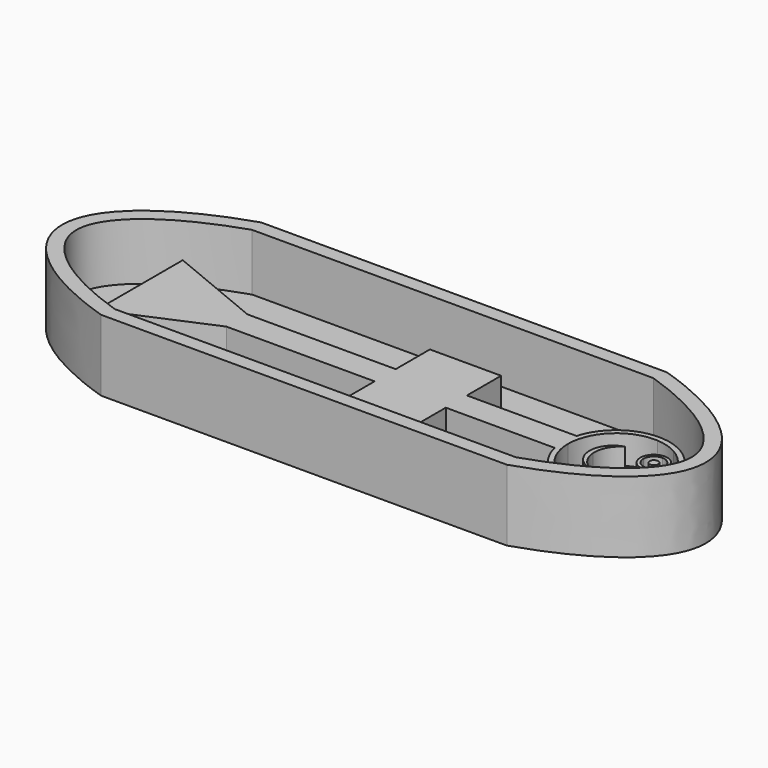
from build123d import *

# Parameters (mm, degrees)
F1_DEPTH  = 12.7
F2_T      = -2.54
F3_R      = 9.525
F4_DEPTH  = 5.08
F5_W      = 58.697837091
F5_H      = 4.7092778205
F6_DEPTH  = 5.08
F8_DEPTH  = 5.08
F9_W      = 12.7
F9_H      = 7.62
F10_DEPTH = 5.08


with BuildPart() as f1:
    # F0 (on Top) → F1 (new body)
    with BuildSketch(Plane.XY):
        with BuildLine():
            Line((-36.1903431505, -17.8440727383), (36.1903431505, -17.8440727383))
            add(Edge.make_bspline(
                [(36.1903431505, -17.8440727383), (91.0502120584, 0), (36.1903431505, 17.8440727383)],
                knots=[2.2529388906, 2.2529388906, 2.2529388906, 4.0302464165, 4.0302464165, 4.0302464165], degree=2, weights=[1, 0.6304575787, 1]))
            Line((36.1903431505, 17.8440727383), (-36.1903431505, 17.8440727383))
            add(Edge.make_bspline(
                [(-36.1903431505, 17.8440727383), (-91.0502120584, 0), (-36.1903431505, -17.8440727383)],
                knots=[5.3945315442, 5.3945315442, 5.3945315442, 7.1718390701, 7.1718390701, 7.1718390701], degree=2, weights=[1, 0.6304575787, 1]))
        make_face()
    extrude(amount=F1_DEPTH)

    # F2
    f2_openings = [f1.faces().sort_by_distance(p)[0] for p in [
        (0, 0, 12.7),
    ]]
    offset(amount=F2_T, openings=f2_openings, kind=Kind.INTERSECTION)

    # F3 (on face) → F4 (join)
    with BuildSketch(Plane.XY.offset(2.54)):
        with Locations((41.4168211738, 0)):
            Circle(F3_R)
        with BuildLine():
            ThreePointArc((49.4494469318, 3.058769096), (49.8702806957, 1.5550456789), (50.0121190134, 0))
            ThreePointArc((50.0121190134, 0), (49.8638586871, -1.5895603794), (49.4241923942, -3.1242840923))
            ThreePointArc((49.4241923942, -3.1242840923), (47.9319414134, -5.6064563866), (45.6999853593, -7.452090278))
            ThreePointArc((45.6999853593, -7.452090278), (43.8819573516, -8.2342120799), (41.9332322253, -8.57977066))
            ThreePointArc((41.9332322253, -8.57977066), (35.5244346388, -6.2577093152), (32.8215233342, 0))
            ThreePointArc((32.8215233342, 0), (35.5244346388, 6.2577093152), (41.9332322253, 8.57977066))
            ThreePointArc((41.9332322253, 8.57977066), (43.8819573516, 8.2342120799), (45.6999853593, 7.452090278))
            ThreePointArc((45.6999853593, 7.452090278), (47.9547863187, 5.5797989853), (49.4494469318, 3.058769096))
        make_face(mode=Mode.SUBTRACT)
        with BuildLine():
            Line((45.6999853593, 4.9295564949), (45.6999853593, 5.471769096))
            ThreePointArc((45.6999853593, 5.471769096), (43.9937366963, 4.765017759), (43.2869853593, 3.058769096))
            Line((43.2869853593, 3.058769096), (43.8291979604, 3.058769096))
            ThreePointArc((43.8291979604, 3.058769096), (44.3771389034, 4.381615552), (45.6999853593, 4.9295564949))
        make_face()
        with BuildLine():
            Line((47.5707727582, 3.058769096), (48.1129853593, 3.058769096))
            ThreePointArc((48.1129853593, 3.058769096), (47.4062340223, 4.765017759), (45.6999853593, 5.471769096))
            Line((45.6999853593, 5.471769096), (45.6999853593, 4.9295564949))
            ThreePointArc((45.6999853593, 4.9295564949), (47.0228318152, 4.381615552), (47.5707727582, 3.058769096))
        make_face()
        with BuildLine():
            ThreePointArc((45.6999853593, 0.645769096), (47.4062340223, 1.352520433), (48.1129853593, 3.058769096))
            Line((48.1129853593, 3.058769096), (47.5707727582, 3.058769096))
            ThreePointArc((47.5707727582, 3.058769096), (47.0228318152, 1.7359226401), (45.6999853593, 1.1879816971))
            Line((45.6999853593, 1.1879816971), (45.6999853593, 0.645769096))
        make_face()
        with BuildLine():
            ThreePointArc((43.2869853593, 3.058769096), (43.9937366963, 1.352520433), (45.6999853593, 0.645769096))
            Line((45.6999853593, 0.645769096), (45.6999853593, 1.1879816971))
            ThreePointArc((45.6999853593, 1.1879816971), (44.3771389034, 1.7359226401), (43.8291979604, 3.058769096))
            Line((43.8291979604, 3.058769096), (43.2869853593, 3.058769096))
        make_face()
        with BuildLine():
            Line((45.6999853593, -1.2536188461), (45.6999853593, -0.7113778659))
            ThreePointArc((45.6999853593, -0.7113778659), (43.9800014557, -1.4105307746), (43.2657123098, -3.1242840923))
            Line((43.2657123098, -3.1242840923), (43.8079261098, -3.1242840923))
            ThreePointArc((43.8079261098, -3.1242840923), (44.363409364, -1.7939385858), (45.6999853593, -1.2536188461))
        make_face()
        with BuildLine():
            ThreePointArc((43.2657123098, -3.1242840923), (43.9800014557, -4.8380374101), (45.6999853593, -5.5371903187))
            Line((45.6999853593, -5.5371903187), (45.6999853593, -4.9949493386))
            ThreePointArc((45.6999853593, -4.9949493386), (44.363409364, -4.4546295989), (43.8079261098, -3.1242840923))
            Line((43.8079261098, -3.1242840923), (43.2657123098, -3.1242840923))
        make_face()
        with BuildLine():
            ThreePointArc((45.6999853593, -5.5371903187), (47.3924656276, -4.8229949464), (48.0917123098, -3.1242840923))
            Line((48.0917123098, -3.1242840923), (47.5494985098, -3.1242840923))
            ThreePointArc((47.5494985098, -3.1242840923), (47.0090578163, -4.4395870382), (45.6999853593, -4.9949493386))
            Line((45.6999853593, -4.9949493386), (45.6999853593, -5.5371903187))
        make_face()
        with BuildLine():
            Line((47.5494985098, -3.1242840923), (48.0917123098, -3.1242840923))
            ThreePointArc((48.0917123098, -3.1242840923), (47.3924656276, -1.4255732382), (45.6999853593, -0.7113778659))
            Line((45.6999853593, -0.7113778659), (45.6999853593, -1.2536188461))
            ThreePointArc((45.6999853593, -1.2536188461), (47.0090578163, -1.8089811465), (47.5494985098, -3.1242840923))
        make_face()
        with BuildLine():
            Line((45.6999853593, 3.058769096), (46.4619853593, 3.058769096))
            ThreePointArc((46.4619853593, 3.058769096), (46.2388007265, 3.5975844633), (45.6999853593, 3.820769096))
            Line((45.6999853593, 3.820769096), (45.6999853593, 3.058769096))
        make_face()
        with BuildLine():
            Line((45.6999853593, 3.058769096), (45.6999853593, 3.820769096))
            ThreePointArc((45.6999853593, 3.820769096), (45.161169992, 3.5975844633), (44.9379853593, 3.058769096))
            Line((44.9379853593, 3.058769096), (45.6999853593, 3.058769096))
        make_face()
        with BuildLine():
            ThreePointArc((44.9379853593, 3.058769096), (45.161169992, 2.5199537288), (45.6999853593, 2.296769096))
            Line((45.6999853593, 2.296769096), (45.6999853593, 3.058769096))
            Line((45.6999853593, 3.058769096), (44.9379853593, 3.058769096))
        make_face()
        with BuildLine():
            ThreePointArc((45.6999853593, 2.296769096), (46.2388007265, 2.5199537288), (46.4619853593, 3.058769096))
            Line((46.4619853593, 3.058769096), (45.6999853593, 3.058769096))
            Line((45.6999853593, 3.058769096), (45.6999853593, 2.296769096))
        make_face()
        with BuildLine():
            Line((45.6999853593, -3.1242840923), (46.4407123098, -3.1242840923))
            ThreePointArc((46.4407123098, -3.1242840923), (46.2249970632, -2.5930431224), (45.6999853593, -2.3625810942))
            Line((45.6999853593, -2.3625810942), (45.6999853593, -3.1242840923))
        make_face()
        with BuildLine():
            ThreePointArc((45.6999853593, -3.8859870905), (46.2249970632, -3.6555250623), (46.4407123098, -3.1242840923))
            Line((46.4407123098, -3.1242840923), (45.6999853593, -3.1242840923))
            Line((45.6999853593, -3.1242840923), (45.6999853593, -3.8859870905))
        make_face()
        with BuildLine():
            ThreePointArc((44.9167123098, -3.1242840923), (45.1474713399, -3.6705688458), (45.6999853593, -3.8859870905))
            Line((45.6999853593, -3.8859870905), (45.6999853593, -3.1242840923))
            Line((45.6999853593, -3.1242840923), (44.9167123098, -3.1242840923))
        make_face()
        with BuildLine():
            Line((45.6999853593, -3.1242840923), (45.6999853593, -2.3625810942))
            ThreePointArc((45.6999853593, -2.3625810942), (45.1474713399, -2.5779993389), (44.9167123098, -3.1242840923))
            Line((44.9167123098, -3.1242840923), (45.6999853593, -3.1242840923))
        make_face()
        with BuildLine():
            Line((36.4539885102, 0), (37.2883511223, 0))
            ThreePointArc((37.2883511223, 0), (37.8159306178, 2.4743182211), (39.5707897842, 4.2966958135))
            ThreePointArc((39.5707897842, 4.2966958135), (37.2343782043, 2.7127130848), (36.4539885102, 0))
        make_face()
        with BuildLine():
            ThreePointArc((39.7878214717, -3.7877704017), (38.0391965115, -2.2230921205), (37.2883511223, 0))
            Line((37.2883511223, 0), (36.4539885102, 0))
            ThreePointArc((36.4539885102, 0), (37.4781151741, -2.4596412133), (39.7878214717, -3.7877704017))
        make_face()
    extrude(amount=F4_DEPTH)

    # F5 (on face) → F6 (join)
    with BuildSketch(Plane.XY.offset(2.54)):
        with Locations((2.9075952818, 0.2558005772)):
            Rectangle(F5_W, F5_H)
    extrude(amount=F6_DEPTH)

    # F7 (on face) → F8 (join)
    with BuildSketch(Plane.XY.offset(2.54)):
        Polygon((-26.4413232637, -2.098838333), (-43.6986163259, -7.7735553496), (-43.6986163259, -9.5117790624), align=None)
        Polygon((-26.4413232637, -2.098838333), (-26.4413232637, 2.6104394875), (-43.6986163259, 9.7535261884), (-43.6986163259, -7.7735553496), align=None)
    extrude(amount=F8_DEPTH)

    # F9 (on face) → F10 (join)
    with BuildSketch(Plane.XY.offset(2.54)):
        with Locations((6.35, 6.4204394875)):
            Rectangle(F9_W, F9_H)
        with Locations((6.35, -5.908838333)):
            Rectangle(F9_W, F9_H)
    extrude(amount=F10_DEPTH)


solid = f1.part
